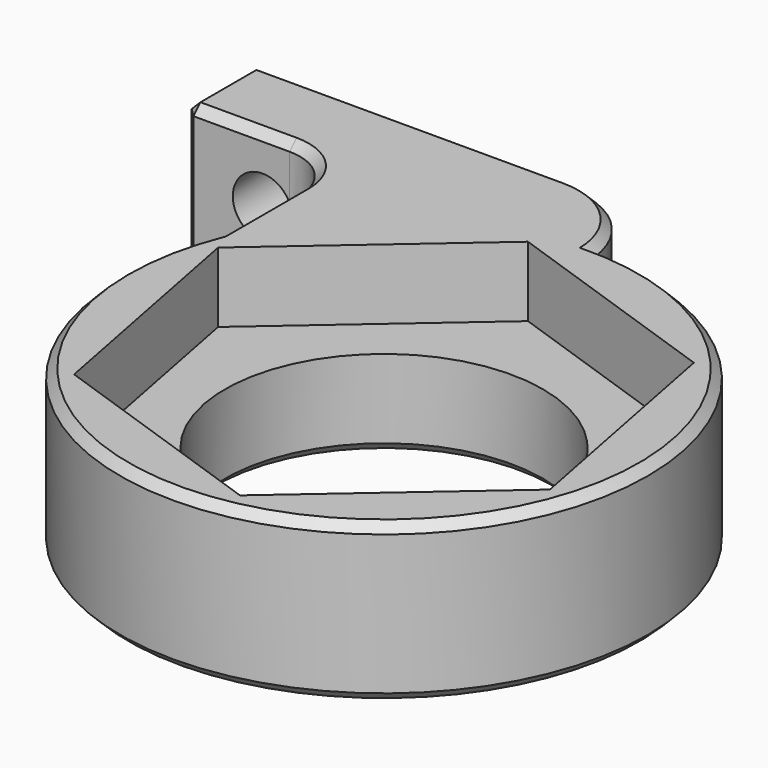
from build123d import *

# Parameters (mm, degrees)
F0_R     = 9.1
F1_DEPTH = 9
F2_SIZE  = 0.5
F3_R     = 1.7
F4_DEPTH = 5.0047524467
F5_R     = 9.1
F6_DEPTH = 4


# Not quite as in the source:
# - a feature names something its author has since deleted; it is built from what else it names


with BuildPart() as f1:
    # F0 (on Top) → F1 (new body)
    with BuildSketch(Plane.XY):
        with BuildLine():
            Line((-14, 11.0595270927), (-14, 5.2172651566))
            ThreePointArc((-14, 5.2172651566), (8.443285949, -12.9592956308), (0, 14.6595270927))
            ThreePointArc((0, 14.6595270927), (-1.647244668, 17.8011844795), (-4.9638694584, 19.0595270927))
            Line((-4.9638694584, 19.0595270927), (-23, 19.0595270927))
            Line((-23, 19.0595270927), (-23, 14.0595270927))
            Line((-23, 14.0595270927), (-17, 14.0595270927))
            ThreePointArc((-17, 14.0595270927), (-14.8786796564, 13.1808474363), (-14, 11.0595270927))
        make_face()
        with Locations((0, -0.4404729073)):
            Circle(F0_R, mode=Mode.SUBTRACT)
    extrude(amount=F1_DEPTH)

    # F2
    f2_edges = [f1.edges().sort_by_distance(p)[0] for p in [
        (-23, 16.559527, 0),
        (-20, 14.059527, 0),
        (-14.87868, 13.180847, 0),
        (-14, 8.138396, 0),
        (8.443286, -12.959296, 0),
        (-1.647245, 17.801184, 0),
        (-13.981935, 19.059527, 0),
        (-9.1, -0.440473, 0),
        (8.443286, -12.959296, 9),
        (-14, 8.138396, 9),
        (-20, 14.059527, 9),
        (-14.87868, 13.180847, 9),
        (-23, 16.559527, 9),
        (-13.981935, 19.059527, 9),
        (-1.647245, 17.801184, 9),
        (-23, 14.059527, 4.5),
    ]]
    chamfer(f2_edges, length=F2_SIZE)

    # F3 (on face) → F4 (cut, through all)
    with BuildSketch(Plane(origin=(0, 19.0595270927, 0), x_dir=(-1, 0, 0), z_dir=(0, 1, 0))):
        with Locations((18.55, 5.2)):
            Circle(F3_R)
    extrude(amount=-F4_DEPTH, mode=Mode.SUBTRACT)

    # F5 (on face) → F6 (cut)
    with BuildSketch(Plane.XY.offset(9)):
        Polygon((-10.4585305038, -9.5299800281), (2.6424788226, -14.0425795703), (13.1010093265, -4.9530724494), (10.4585305038, 8.6490342136), (-2.6424788226, 13.1616337557), (-13.1010093265, 4.0721266349), align=None)
        with Locations((0, -0.4404729073)):
            Circle(F5_R, mode=Mode.SUBTRACT)
    extrude(amount=-F6_DEPTH, mode=Mode.SUBTRACT)


solid = f1.part
